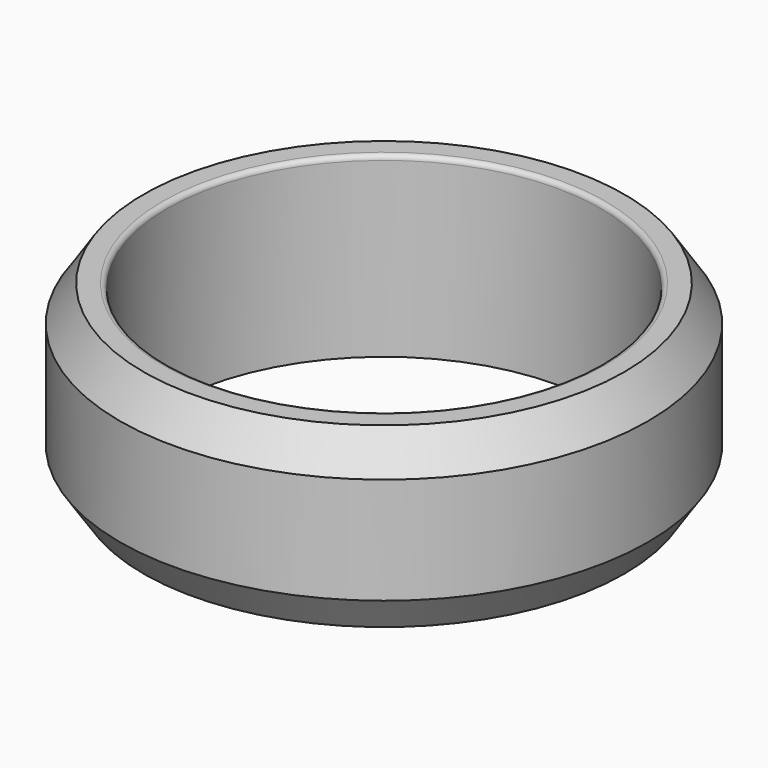
from build123d import *

# Parameters (mm, degrees)
F0_R       = 11.15
F0_R_2     = 9.15
F1_DEPTH   = 7.5
F2_SIZE2   = 1.5
F2_SIZE    = 1
F2_2_SIZE2 = 1.5
F2_2_SIZE  = 1
F3_R       = 0.2


# Not quite as in the source:
# - a feature names something its author has since deleted; it is built from what else it names


with BuildPart() as f1:
    # F0 (on Top) → F1 (new body)
    with BuildSketch(Plane.XY):
        Circle(F0_R)
        Circle(F0_R_2, mode=Mode.SUBTRACT)
    extrude(amount=F1_DEPTH)

    # F2
    f2_edges = [f1.edges().sort_by_distance(p)[0] for p in [
        (-11.15, 0, 7.5),
    ]]
    f2_side = f1.faces().sort_by_distance((-10.83463, 0, 7.5))[0]
    chamfer(f2_edges, length=F2_SIZE, length2=F2_SIZE2, reference=f2_side)

    # F2#2
    f2_2_edges = [f1.edges().sort_by_distance(p)[0] for p in [
        (-11.15, 0, 0),
    ]]
    f2_2_side = f1.faces().sort_by_distance((-10.83463, 0, 0))[0]
    chamfer(f2_2_edges, length=F2_2_SIZE, length2=F2_2_SIZE2, reference=f2_2_side)

    # F3
    f3_edges = [f1.edges().sort_by_distance(p)[0] for p in [
        (-9.15, 0, 7.5),
    ]]
    fillet(f3_edges, radius=F3_R)


solid = f1.part
